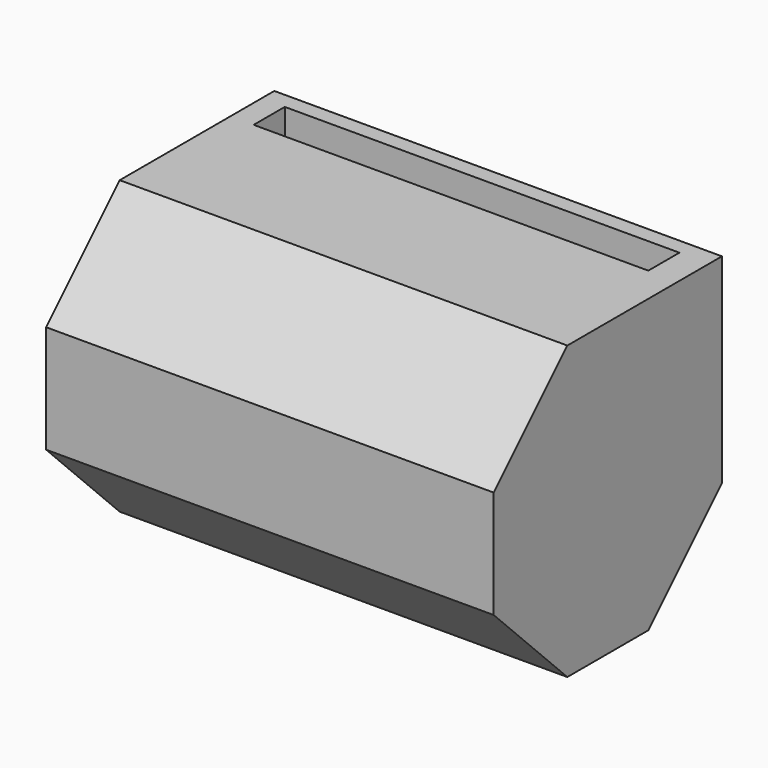
from build123d import *

# Parameters (mm, degrees)
F1_DEPTH = 39.37
F2_SIZE  = 12.7
F3_W     = 54.4642563909
F3_H     = 5.3648606408
F4_DEPTH = 5.588
F5_T     = -2.54


# Not quite as in the source:
# - a shell that OpenCascade refuses in one call is made with other operations: the cavity is built on its own and cut out


with BuildPart() as f1:
    # F0 (on Front) → F1 (new body)
    with BuildSketch(Plane.XZ):
        Polygon((-33.8817872107, 27.0782150328), (-33.8817872107, -13.1989289075), (27.8946403414, -13.1989289075), (27.8946403414, 27.0782150328), (0, 27.0782150328), (-9.9332146347, 27.0782150328), align=None)
    extrude(amount=F1_DEPTH)

    # F2
    f2_edges = [f1.edges().sort_by_distance(p)[0] for p in [
        (-2.993573, -39.37, -13.198929),
        (-2.993573, -39.37, 27.078215),
        (-2.993573, 0, -13.198929),
    ]]
    chamfer(f2_edges, length=F2_SIZE)

    # F3 (on face) → F4 (cut)
    with BuildSketch(Plane.XY.offset(27.0782150328)):
        with Locations((-3.4423777834, -4.8837963259)):
            Rectangle(F3_W, F3_H)
    extrude(amount=-F4_DEPTH, mode=Mode.SUBTRACT)

    # F5: a shell. OpenCascade refuses it in one call, so the cavity is built on its own and cut out:
    # the body offset inwards by the wall thickness, plus a prism from it out through each open face.
    f5_core = offset(f1.part, amount=F5_T, kind=Kind.INTERSECTION, mode=Mode.PRIVATE)
    f5_exits = [f5_core.faces().sort_by_distance(p)[0] for p in [
        (-2.993573, -6.323113, 18.950215),
    ]]
    add(f5_core, mode=Mode.SUBTRACT)
    extrude(f5_exits, amount=-F5_T, mode=Mode.SUBTRACT)


solid = f1.part
